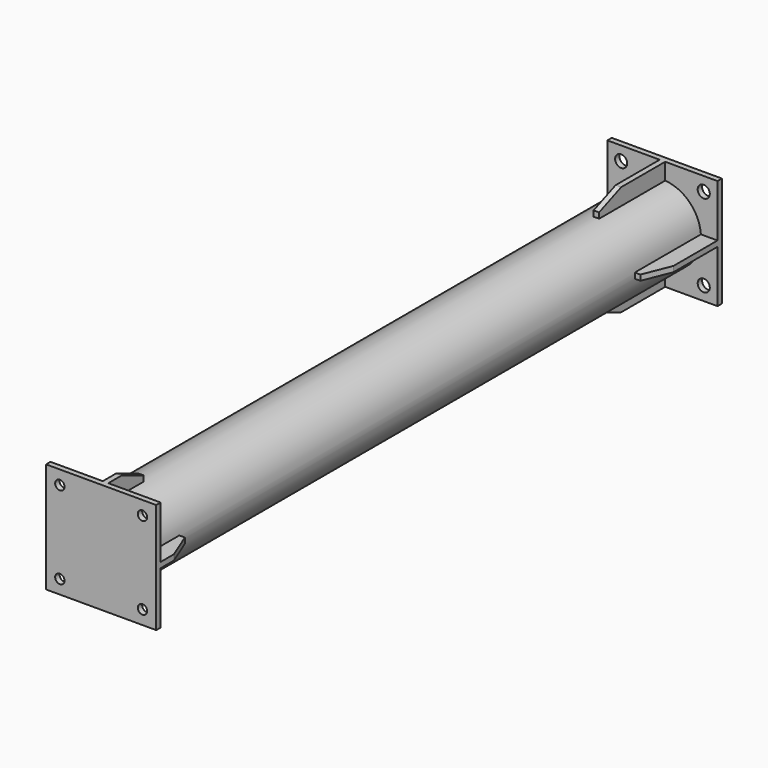
from build123d import *

# Parameters (mm, degrees)
F0_R          = 70
F0_R_2        = 65
F1_DEPTH      = 1264
F2_W          = 200
F2_H          = 200
F2_R          = 11
F3_DEPTH      = 10
F4_W          = 30.1787997812
F4_H          = 10
F4_W_2        = 10
F4_H_2        = 30.1787997812
F5_DEPTH      = 150
F6_T1_DEPTH   = 269.311363913
F6_T3_DEPTH   = 269.311363913
F6_T8_DEPTH   = 269.311363913
F6_S9_R       = 70
F6_T10_DEPTH  = 139
F8_W          = 200
F8_H          = 200
F8_R          = 8.5
F9_DEPTH      = 10
F10_W         = 10
F10_H         = 30.1787997812
F10_W_2       = 30.1787997812
F10_H_2       = 10
F11_DEPTH     = 80
F12_T1_DEPTH  = 269.311363913
F12_T3_DEPTH  = 269.311363913
F12_T8_DEPTH  = 269.311363913
F12_S9_R      = 70
F12_T10_DEPTH = 139
F12_T14_DEPTH = 269.311363913
F12_S15_R     = 70
F12_T16_DEPTH = 139


# Not quite as in the source:
# - a fillet or chamfer that OpenCascade refuses, or shapes differently, is made with other operations: its cross-section is extruded or revolved along the edge and cut away or added


with BuildPart() as f1:
    # F0 (on Front) → F1 (new body)
    with BuildSketch(Plane.XZ):
        Circle(F0_R)
        Circle(F0_R_2, mode=Mode.SUBTRACT)
    extrude(amount=F1_DEPTH)

    # F2 (on Front) → F3 (join)
    with BuildSketch(Plane.XZ):
        Rectangle(F2_W, F2_H)
        with Locations((-75, -75)):
            Circle(F2_R, mode=Mode.SUBTRACT)
        with Locations((75, -75)):
            Circle(F2_R, mode=Mode.SUBTRACT)
        with Locations((-75, 75)):
            Circle(F2_R, mode=Mode.SUBTRACT)
        with Locations((75, 75)):
            Circle(F2_R, mode=Mode.SUBTRACT)
    extrude(amount=-F3_DEPTH)

    # F4 (on Front) → F5 (join)
    with BuildSketch(Plane.XZ):
        with Locations((-84.9106001094, 0)):
            Rectangle(F4_W, F4_H)
        with Locations((0, 84.9106001094)):
            Rectangle(F4_W_2, F4_H_2)
        with Locations((84.9106001094, 0)):
            Rectangle(F4_W, F4_H)
        with Locations((0, -84.9106001094)):
            Rectangle(F4_W_2, F4_H_2)
    extrude(amount=F5_DEPTH)

    # F6: chamfer of 50 x 20 on 4 edges, made by hand

    # F6_s2 → F6_t1 (cut)
    with BuildSketch(Plane.YZ.offset(-134.6556819565)):
        Polygon((-100, 100), (-150, 80), (-150, 100), align=None)
        Polygon((-100, -100), (-150, -80), (-150, -100), align=None)
    extrude(amount=F6_T1_DEPTH, mode=Mode.SUBTRACT)

    # F6_s4 → F6_t3 (cut)
    with BuildSketch(Plane.XY.offset(-134.6556819565)):
        Polygon((100, -100), (80, -150), (100, -150), align=None)
    extrude(amount=F6_T3_DEPTH, mode=Mode.SUBTRACT)


with BuildPart() as f6_tool6:
    # F6_s7 → F6_t8 (new body)
    with BuildSketch(Plane.XY.offset(134.6556819565)):
        Polygon((-100, -130), (-50, -150), (-100, -150), align=None)
    extrude(amount=-F6_T8_DEPTH)

    # F6_s9 → F6_t10 (cut, symmetric)
    with BuildSketch(Plane.XZ.offset(140)):
        Circle(F6_S9_R)
    extrude(amount=F6_T10_DEPTH, both=True, mode=Mode.SUBTRACT)


with BuildPart() as f1_1:
    add(f1.part)

    # F6_t5: cut F6_tool6
    add(f6_tool6.part, mode=Mode.SUBTRACT)

    # F8 (on offset) → F9 (join)
    with BuildSketch(Plane.XZ.offset(1264)):
        Rectangle(F8_W, F8_H)
        with Locations((-75, -75)):
            Circle(F8_R, mode=Mode.SUBTRACT)
        with Locations((75, -75)):
            Circle(F8_R, mode=Mode.SUBTRACT)
        with Locations((-75, 75)):
            Circle(F8_R, mode=Mode.SUBTRACT)
        with Locations((75, 75)):
            Circle(F8_R, mode=Mode.SUBTRACT)
    extrude(amount=F9_DEPTH)

    # F10 (on face) → F11 (join)
    with BuildSketch(Plane(origin=(0, -1264, 0), x_dir=(-1, 0, 0), z_dir=(0, 1, 0))):
        with Locations((0, 84.9106001094)):
            Rectangle(F10_W, F10_H)
        with Locations((84.9106001094, 0)):
            Rectangle(F10_W_2, F10_H_2)
        with Locations((0, -84.9106001094)):
            Rectangle(F10_W, F10_H)
        with Locations((-84.9106001094, 0)):
            Rectangle(F10_W_2, F10_H_2)
    extrude(amount=F11_DEPTH)

    # F12: chamfer of 20 x 50 on 4 edges, made by hand

    # F12_s2 → F12_t1 (cut)
    with BuildSketch(Plane.YZ.offset(-134.6556819565)):
        Polygon((-1234, 100), (-1184, 80), (-1184, 100), align=None)
    extrude(amount=F12_T1_DEPTH, mode=Mode.SUBTRACT)

    # F12_s4 → F12_t3 (cut)
    with BuildSketch(Plane.XY.offset(-134.6556819565)):
        Polygon((100, -1234), (80, -1184), (100, -1184), align=None)
    extrude(amount=F12_T3_DEPTH, mode=Mode.SUBTRACT)


with BuildPart() as f12_tool6:
    # F12_s7 → F12_t8 (new body)
    with BuildSketch(Plane.XY.offset(-134.6556819565)):
        Polygon((-100, -1204), (-50, -1184), (-100, -1184), align=None)
    extrude(amount=F12_T8_DEPTH)

    # F12_s9 → F12_t10 (cut, symmetric)
    with BuildSketch(Plane.XZ.offset(1194)):
        Circle(F12_S9_R)
    extrude(amount=F12_T10_DEPTH, both=True, mode=Mode.SUBTRACT)


with BuildPart() as f1_2:
    add(f1_1.part)

    # F12_t5: cut F12_tool6
    add(f12_tool6.part, mode=Mode.SUBTRACT)


with BuildPart() as f12_tool12:
    # F12_s13 → F12_t14 (new body)
    with BuildSketch(Plane.YZ.offset(134.6556819565)):
        Polygon((-1204, -100), (-1184, -50), (-1184, -100), align=None)
    extrude(amount=-F12_T14_DEPTH)

    # F12_s15 → F12_t16 (cut, symmetric)
    with BuildSketch(Plane.XZ.offset(1194)):
        Circle(F12_S15_R)
    extrude(amount=F12_T16_DEPTH, both=True, mode=Mode.SUBTRACT)


with BuildPart() as f1_3:
    add(f1_2.part)

    # F12_t11: cut F12_tool12
    add(f12_tool12.part, mode=Mode.SUBTRACT)


solid = f1_3.part
